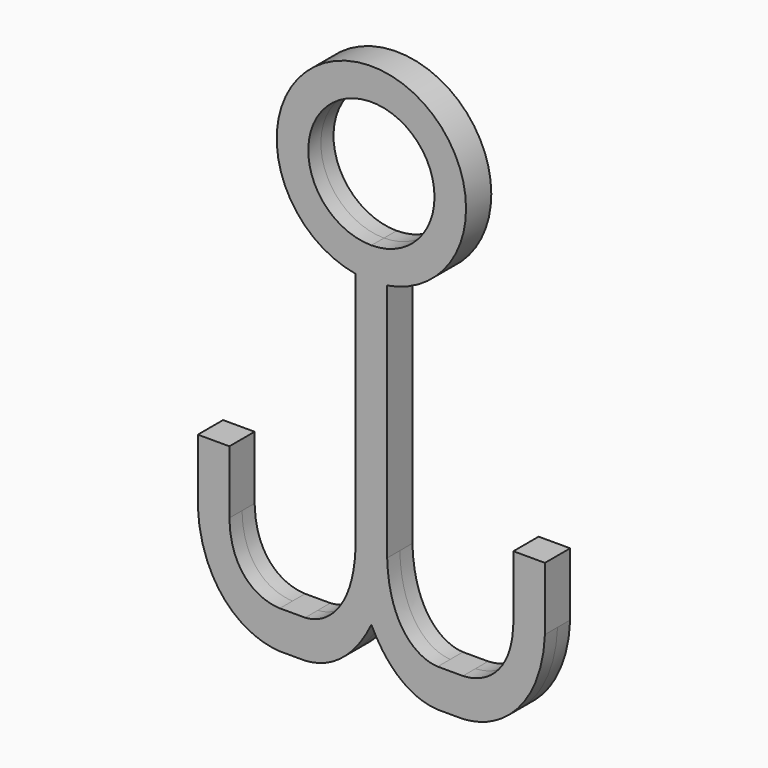
from build123d import *

# Parameters (mm, degrees)
F0_W     = 25.4
F0_H     = 38.1
F0_W_2   = 31.75
F0_H_2   = 63.5
F1_DEPTH = 15.875


with BuildPart() as f1:
    # F0 (on Front) → F1 (new body, symmetric)
    with BuildSketch(Plane.XZ):
        with BuildLine():
            Line((-15.875, -103.8391655019), (-15.875, -345.1981674205))
            Line((-15.875, -345.1981674205), (0, -345.1981674205))
            Line((0, -345.1981674205), (0, -105.1713989452))
            ThreePointArc((0, -105.1713989452), (-7.9654012916, -104.8377562407), (-15.875, -103.8391655019))
        make_face()
        with BuildLine():
            add(Edge.make_bspline(
                [(0, -409.482145582), (-10.3991862171, -388.0156164118), (-15.7271620535, -363.9765002128), (-15.875, -345.1981674205)],
                knots=[81.5477604067, 81.5477604067, 81.5477604067, 81.5477604067, 143.8364349915, 143.8364349915, 143.8364349915, 143.8364349915], degree=3))
            add(Edge.make_bspline(
                [(-66.675, -424.8878848455), (-44.6960218251, -423.8382875919), (-17.5926852971, -402.3276865482), (-15.875, -345.1981674205)],
                knots=[0, 0, 0, 0, 94.5044499655, 94.5044499655, 94.5044499655, 94.5044499655], degree=3))
            Line((-66.675, -424.8878848455), (-66.675, -462.9878848455))
            add(Edge.make_bspline(
                [(-66.675, -462.9878848455), (-35.9209941881, -461.2803468487), (-13.6145190391, -437.5859283193), (0, -409.482145582)],
                knots=[0, 0, 0, 0, 81.5477604067, 81.5477604067, 81.5477604067, 81.5477604067], degree=3))
        make_face()
        with BuildLine():
            Line((0, -345.1981674205), (-15.875, -345.1981674205))
            add(Edge.make_bspline(
                [(0, -409.482145582), (-10.3991862171, -388.0156164118), (-15.7271620535, -363.9765002128), (-15.875, -345.1981674205)],
                knots=[81.5477604067, 81.5477604067, 81.5477604067, 81.5477604067, 143.8364349915, 143.8364349915, 143.8364349915, 143.8364349915], degree=3))
            add(Edge.make_bspline(
                [(0, -409.482145582), (10.3991862171, -388.0156164118), (15.7271620535, -363.9765002128), (15.875, -345.1981674205)],
                knots=[81.5477604067, 81.5477604067, 81.5477604067, 81.5477604067, 143.8364349915, 143.8364349915, 143.8364349915, 143.8364349915], degree=3))
            Line((15.875, -345.1981674205), (0, -345.1981674205))
        make_face()
        with BuildLine():
            Line((0, -105.1713989452), (0, -345.1981674205))
            Line((0, -345.1981674205), (15.875, -345.1981674205))
            Line((15.875, -345.1981674205), (15.875, -103.8391655019))
            ThreePointArc((15.875, -103.8391655019), (7.9654012916, -104.8377562407), (0, -105.1713989452))
        make_face()
        with BuildLine():
            ThreePointArc((95.25, -9.9213989452), (-61.483610621, 62.8269902123), (-15.875, -103.8391655019))
            Line((-15.875, -103.8391655019), (-15.875, -91.1981674205))
            Line((-15.875, -91.1981674205), (0, -91.1981674205))
            Line((0, -91.1981674205), (15.875, -91.1981674205))
            Line((15.875, -91.1981674205), (15.875, -103.8391655019))
            ThreePointArc((15.875, -103.8391655019), (72.7483891574, -71.4050095662), (95.25, -9.9213989452))
        make_face()
        with BuildLine():
            ThreePointArc((63.5, -9.9213989452), (44.9012806053, -54.8226795505), (0, -73.4213989452))
            ThreePointArc((0, -73.4213989452), (-44.9012806053, 34.9798816602), (63.5, -9.9213989452))
        make_face(mode=Mode.SUBTRACT)
        with BuildLine():
            Line((-15.875, -91.1981674205), (-15.875, -103.8391655019))
            ThreePointArc((-15.875, -103.8391655019), (-7.9654012916, -104.8377562407), (0, -105.1713989452))
            Line((0, -105.1713989452), (0, -91.1981674205))
            Line((0, -91.1981674205), (-15.875, -91.1981674205))
        make_face()
        with Locations((-79.375, -443.9378848455)):
            Rectangle(F0_W, F0_H)
        with BuildLine():
            add(Edge.make_bspline(
                [(0, -409.482145582), (10.3991862171, -388.0156164118), (15.7271620535, -363.9765002128), (15.875, -345.1981674205)],
                knots=[81.5477604067, 81.5477604067, 81.5477604067, 81.5477604067, 143.8364349915, 143.8364349915, 143.8364349915, 143.8364349915], degree=3))
            add(Edge.make_bspline(
                [(66.675, -462.9878848455), (35.9209941881, -461.2803468487), (13.6145190391, -437.5859283193), (0, -409.482145582)],
                knots=[0, 0, 0, 0, 81.5477604067, 81.5477604067, 81.5477604067, 81.5477604067], degree=3))
            Line((66.675, -462.9878848455), (66.675, -424.8878848455))
            add(Edge.make_bspline(
                [(66.675, -424.8878848455), (44.6960218251, -423.8382875919), (17.5926852971, -402.3276865482), (15.875, -345.1981674205)],
                knots=[0, 0, 0, 0, 94.5044499655, 94.5044499655, 94.5044499655, 94.5044499655], degree=3))
        make_face()
        with BuildLine():
            Line((0, -91.1981674205), (0, -105.1713989452))
            ThreePointArc((0, -105.1713989452), (7.9654012916, -104.8377562407), (15.875, -103.8391655019))
            Line((15.875, -103.8391655019), (15.875, -91.1981674205))
            Line((15.875, -91.1981674205), (0, -91.1981674205))
        make_face()
        with BuildLine():
            Line((-92.075, -462.9878848455), (-92.075, -424.8878848455))
            add(Edge.make_bspline(
                [(-142.875, -361.3878848455), (-142.1477283955, -404.0485322475), (-118.0558662534, -423.8382875919), (-92.075, -424.8878848455)],
                knots=[0, 0, 0, 0, 81.3196778154, 81.3196778154, 81.3196778154, 81.3196778154], degree=3))
            Line((-142.875, -361.3878848455), (-174.625, -361.3878848455))
            add(Edge.make_bspline(
                [(-174.625, -361.3878848455), (-172.2625430346, -420.826792717), (-136.5549724221, -460.4062736034), (-92.075, -462.9878848455)],
                knots=[0, 0, 0, 0, 130.9086036134, 130.9086036134, 130.9086036134, 130.9086036134], degree=3))
        make_face()
        with Locations((79.375, -443.9378848455)):
            Rectangle(F0_W, F0_H)
        with Locations((-158.75, -329.6378848455)):
            Rectangle(F0_W_2, F0_H_2)
        with BuildLine():
            Line((92.075, -424.8878848455), (92.075, -462.9878848455))
            add(Edge.make_bspline(
                [(174.625, -361.3878848455), (172.2625430346, -420.826792717), (136.5549724221, -460.4062736034), (92.075, -462.9878848455)],
                knots=[0, 0, 0, 0, 130.9086036134, 130.9086036134, 130.9086036134, 130.9086036134], degree=3))
            Line((174.625, -361.3878848455), (142.875, -361.3878848455))
            add(Edge.make_bspline(
                [(142.875, -361.3878848455), (142.1477283955, -404.0485322475), (118.0558662534, -423.8382875919), (92.075, -424.8878848455)],
                knots=[0, 0, 0, 0, 81.3196778154, 81.3196778154, 81.3196778154, 81.3196778154], degree=3))
        make_face()
        with Locations((158.75, -329.6378848455)):
            Rectangle(F0_W_2, F0_H_2)
    extrude(amount=F1_DEPTH, both=True)


solid = f1.part
